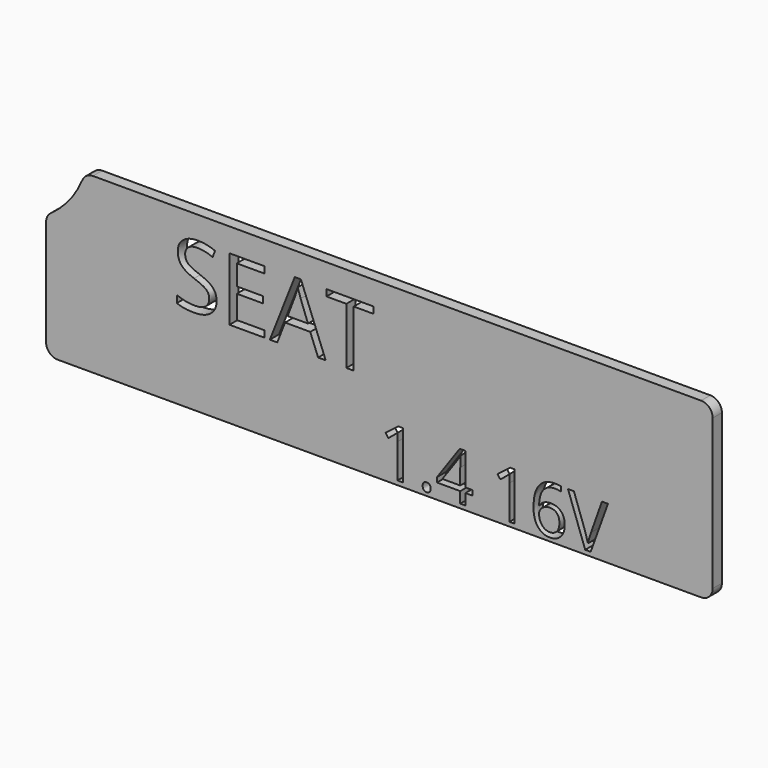
from build123d import *

# Parameters (mm, degrees)
F1_DEPTH     = 2
F2_R         = 2
F3_TEXT_SIZE = 15.2469754943
F4_DEPTH     = 20.3
F5_TEXT_SIZE = 11.5927418746
F6_DEPTH     = 15.8


# Not quite as in the source:
# - Text() gives the source's letters only with a copy of the font that has no kerning and outlines rounded to 1/6400 em; it was checked with that copy


with BuildPart() as f1:
    # F0 (on Front) → F1 (new body)
    with BuildSketch(Plane.XZ):
        with BuildLine():
            Line((55.6108880341, 14.9697586894), (-50.8895312046, 14.9697586894))
            ThreePointArc((-50.8895312046, 14.9697586894), (-53.4909157436, 10.0898455286), (-57.6108880341, 6.401135415))
            Line((-57.6108880341, 6.401135415), (-57.6108880341, -12.9697586894))
            ThreePointArc((-57.6108880341, -12.9697586894), (-57.0251015965, -14.3839722518), (-55.6108880341, -14.9697586894))
            Line((-55.6108880341, -14.9697586894), (55.6108880341, -14.9697586894))
            ThreePointArc((55.6108880341, -14.9697586894), (57.0251015965, -14.3839722518), (57.6108880341, -12.9697586894))
            Line((57.6108880341, -12.9697586894), (57.6108880341, 12.9697586894))
            ThreePointArc((57.6108880341, 12.9697586894), (57.0251015965, 14.3839722518), (55.6108880341, 14.9697586894))
        make_face()
    extrude(amount=F1_DEPTH)

    # F2
    f2_edges = [f1.edges().sort_by_distance(p)[0] for p in [
        (-57.610888, -1, 6.401135),
        (-50.889531, -1, 14.969759),
    ]]
    fillet(f2_edges, radius=F2_R)

    # F3 (on Front) → F4 (cut)
    with BuildSketch(Plane.XZ):
        with Locations((-35.7779809334, 0)):
            Text('SEAT', F3_TEXT_SIZE, font='Open Sans', text_align=(TextAlign.LEFT, TextAlign.BOTTOM))
    extrude(amount=F4_DEPTH, mode=Mode.SUBTRACT)

    # F5 (on Front) → F6 (cut)
    with BuildSketch(Plane.XZ):
        with Locations((0, -14.2439519987)):
            Text('1.4 16V', F5_TEXT_SIZE, font='Open Sans', text_align=(TextAlign.LEFT, TextAlign.BOTTOM))
    extrude(amount=F6_DEPTH, mode=Mode.SUBTRACT)


solid = f1.part
